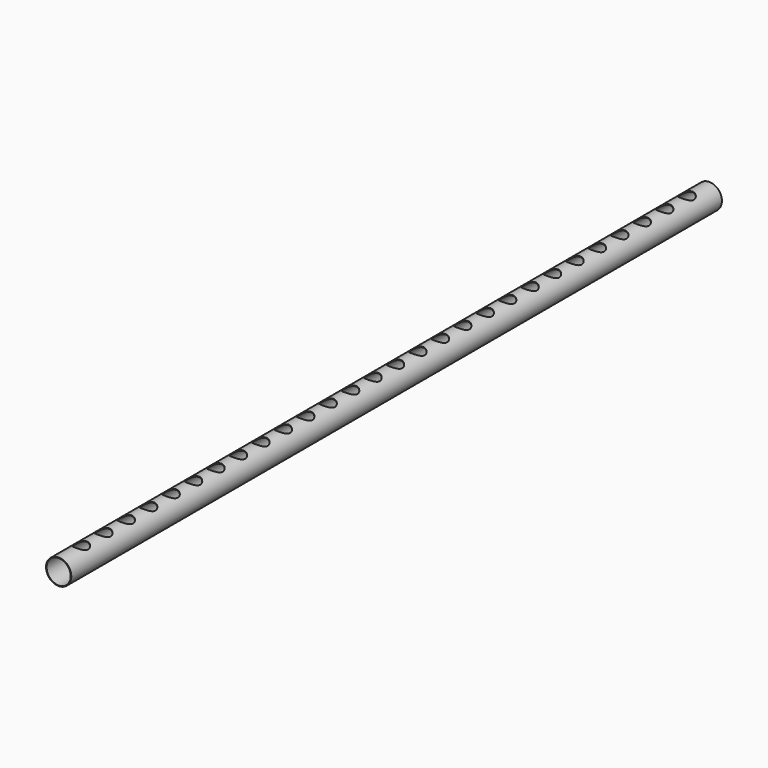
from build123d import *

# Parameters (mm, degrees)
F0_R     = 45
F0_R_2   = 43
F1_DEPTH = 1450
F4_D     = 50
F4_DEPTH = 50
F4_TIP   = 15.0215154757
F6_D     = 0.5
F6_DEPTH = 50
F6_TIP   = 0.1502151548


# Not quite as in the source:
# - a feature names something its author has since deleted; it is built from what else it names


with BuildPart() as f1:
    # F0 (on Front) → F1 (new body, symmetric)
    with BuildSketch(Plane.XZ):
        Circle(F0_R)
        Circle(F0_R_2, mode=Mode.SUBTRACT)
    extrude(amount=F1_DEPTH, both=True)

    # F4
    with Locations(Plane.XY.offset(45)):
        with Locations((0, -1350), (0, -1250), (0, -1150), (0, -1050), (0, -950), (0, -850), (0, -750), (0, -650), (0, -550), (0, -450), (0, -350), (0, -250), (0, -150), (0, -50), (0, 50), (0, 150), (0, 250), (0, 350), (0, 450), (0, 550), (0, 650), (0, 750), (0, 850), (0, 950), (0, 1050), (0, 1150), (0, 1250), (0, 1350)):
            Hole(F4_D / 2, depth=F4_DEPTH)
            with Locations((0, 0, -(F4_DEPTH + F4_TIP / 2))):  # 118° drill point
                Cone(0, F4_D / 2, F4_TIP, mode=Mode.SUBTRACT)

    # F6 (one way)
    with BuildSketch(Plane.XY):
        with Locations((0, 0)):
            Circle(F6_D / 2)
    extrude(amount=-F6_DEPTH, mode=Mode.SUBTRACT)
    with Locations(Plane.XY):
        with Locations((0, 0)):
            with Locations((0, 0, -(F6_DEPTH + F6_TIP / 2))):  # 118° drill point
                Cone(0, F6_D / 2, F6_TIP, mode=Mode.SUBTRACT)


solid = f1.part
